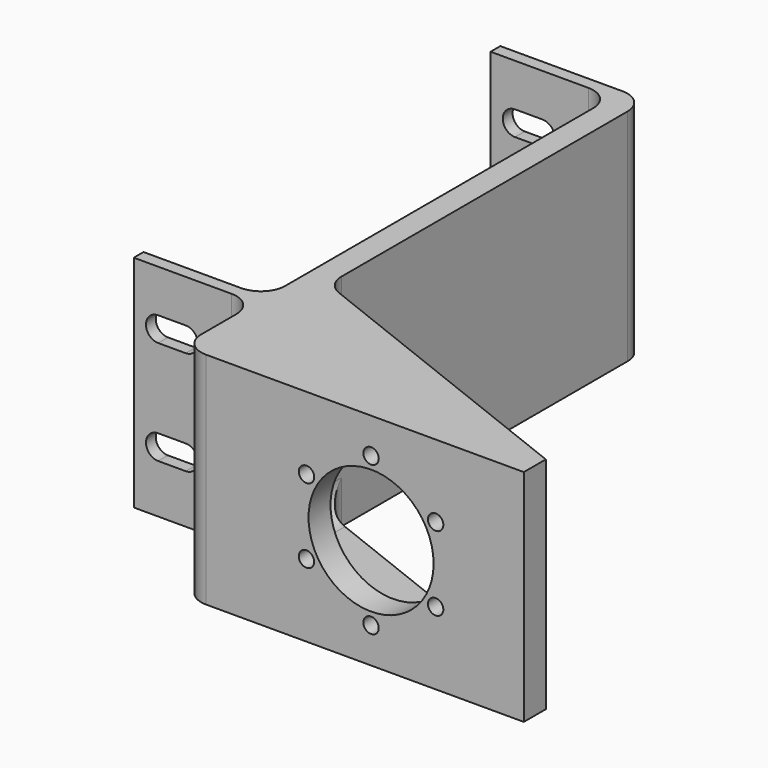
from build123d import *

# Parameters (mm, degrees)
F0_W           = 95.25
F0_H           = 45.72
F1_DEPTH       = 5.08
F2_W           = 2.54
F2_H           = 45.72
F3_DEPTH       = 25.4
F5_DEPTH       = 95.251
F5_DEPTH_BACK  = 163
F8_W           = 71.12
F8_H           = 31.75
F9_DEPTH       = 22.86
F9_DEPTH_BACK  = 22.86
F10_W          = 66.04
F10_H          = 38.1
F11_DEPTH      = 95.251
F11_DEPTH_BACK = 13.589
F13_DEPTH      = 45.721
F13_DEPTH_BACK = 190
F14_R          = 1.6
F14_R_2        = 13
F15_DEPTH      = 19.305
F16_R          = 5.08


# Not quite as in the source:
# - an extrude ends at something that could not be found from the text; its depth is read off the source's solid


with BuildPart() as f1:
    # F0 (on Right) → F1 (new body)
    with BuildSketch(Plane.YZ):
        with Locations((47.625, -22.86)):
            Rectangle(F0_W, F0_H)
    extrude(amount=F1_DEPTH)

    # F2 (on Right) → F3 (join)
    with BuildSketch(Plane.YZ):
        with Locations((93.98, -22.86)):
            Rectangle(F2_W, F2_H)
        with Locations((1.27, -22.86)):
            Rectangle(F2_W, F2_H)
    extrude(amount=-F3_DEPTH)

    # F4 (on Front) → F5 (cut, two sides)
    with BuildSketch(Plane.XZ) as f5_sk:
        with BuildLine():
            Line((-20.32, -13.97), (-14.605, -13.97))
            ThreePointArc((-14.605, -13.97), (-12.065, -11.43), (-14.605, -8.89))
            Line((-14.605, -8.89), (-20.32, -8.89))
            ThreePointArc((-20.32, -8.89), (-22.86, -11.43), (-20.32, -13.97))
        make_face()
        with BuildLine():
            Line((-20.32, -35.56), (-14.605, -35.56))
            ThreePointArc((-14.605, -35.56), (-12.065, -33.02), (-14.605, -30.48))
            Line((-14.605, -30.48), (-20.32, -30.48))
            ThreePointArc((-20.32, -30.48), (-22.86, -33.02), (-20.32, -35.56))
        make_face()
    extrude(amount=-F5_DEPTH, mode=Mode.SUBTRACT)
    extrude(f5_sk.sketch, amount=F5_DEPTH_BACK, mode=Mode.SUBTRACT)

    # F8 (on plane+point) → F9 (join, two sides)
    with BuildSketch(Plane.XY.offset(-22.86)) as f9_sk:
        with Locations((35.56, -3.429)):
            Rectangle(F8_W, F8_H)
    extrude(amount=-F9_DEPTH)
    extrude(f9_sk.sketch, amount=F9_DEPTH_BACK)

    # F10 (on Front) → F11 (cut, two sides)
    with BuildSketch(Plane.XZ) as f11_sk:
        with Locations((38.1, -22.86)):
            Rectangle(F10_W, F10_H)
    extrude(amount=-F11_DEPTH, mode=Mode.SUBTRACT)
    extrude(f11_sk.sketch, amount=F11_DEPTH_BACK, mode=Mode.SUBTRACT)

    # F12 (on Top) → F13 (cut, two sides)
    with BuildSketch(Plane.XY) as f13_sk:
        Polygon((5.08, 12.446), (71.12, -13.589), (71.12, 12.446), align=None)
    extrude(amount=-F13_DEPTH, mode=Mode.SUBTRACT)
    extrude(f13_sk.sketch, amount=F13_DEPTH_BACK, mode=Mode.SUBTRACT)

    # F14 (on Front) → F15 (cut, through all)
    with BuildSketch(Plane.XZ):
        with Locations((39.37, -7.36)):
            Circle(F14_R)
        with Locations((25.9466062413, -15.11)):
            Circle(F14_R)
        with Locations((25.9466062413, -30.61)):
            Circle(F14_R)
        with Locations((39.37, -38.36)):
            Circle(F14_R)
        with Locations((52.7933937587, -30.61)):
            Circle(F14_R)
        with Locations((52.7933937587, -15.11)):
            Circle(F14_R)
        with Locations((39.37, -22.86)):
            Circle(F14_R_2)
    extrude(amount=F15_DEPTH, mode=Mode.SUBTRACT)

    # F16
    f16_edges = [f1.edges().sort_by_distance(p)[0] for p in [
        (0, 92.71, -22.86),
        (0, 2.54, -22.86),
        (0, 0, -22.86),
        (0, -19.304, -22.86),
        (5.08, -13.589, -22.86),
        (5.08, -0.5715, -3.81),
        (5.08, -0.5715, -41.91),
        (5.08, 12.446, -1.905),
        (5.08, 12.446, -43.815),
        (5.08, 95.25, -22.86),
    ]]
    fillet(f16_edges, radius=F16_R)


solid = f1.part
